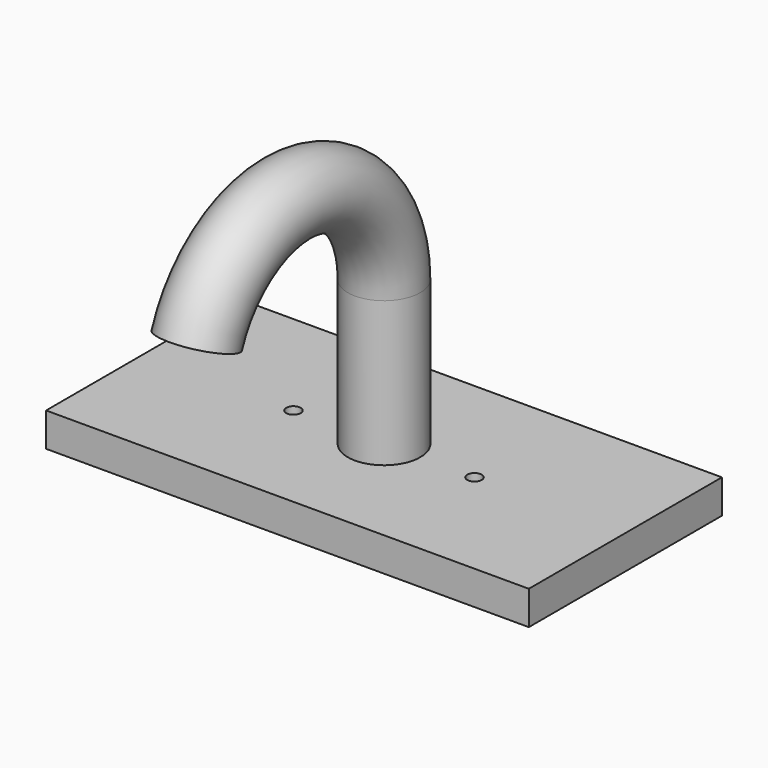
from build123d import *

# Parameters (mm, degrees)
F0_W     = 100
F0_H     = 50
F1_DEPTH = 7
F2_R     = 1.5
F3_DEPTH = 25
F4_R     = 7.5
F5_DEPTH = 30
F4_W     = 5.0690565258
F4_H     = 5.2306629717
F6_R     = 7.5
F7_ANGLE = 160


with BuildPart() as f1:
    # F0 (on Top) → F1 (new body)
    with BuildSketch(Plane.XY):
        Rectangle(F0_W, F0_H)
    extrude(amount=F1_DEPTH)

    # F2 (on face) → F3 (cut)
    with BuildSketch(Plane.XY.offset(7)):
        with Locations((18.7491867621, 0)):
            Circle(F2_R)
        with Locations((-18.7491867621, 0)):
            Circle(F2_R)
    extrude(amount=-F3_DEPTH, mode=Mode.SUBTRACT)


with BuildPart() as f5:
    # F4 (on face) → F5 (new body)
    with BuildSketch(Plane.XY.offset(7)):
        Circle(F4_R)
    extrude(amount=F5_DEPTH)


with BuildPart() as f5b:
    # F4 (on face) → F5, piece 2 (new body)
    with BuildSketch(Plane.XY.offset(7)):
        with Locations((2.5345282629, -22.3846685141)):
            Rectangle(F4_W, F4_H)
    extrude(amount=F5_DEPTH)


with BuildPart() as f7:
    # F6 (on face) → F7 (revolve)
    with BuildSketch(Plane.XY.offset(37)):
        Circle(F6_R)
    revolve(axis=Axis((2.5345282629, -25, 37), (1, 0, 0)), revolution_arc=F7_ANGLE)


solid = Compound([f1.part, f5.part, f7.part])
